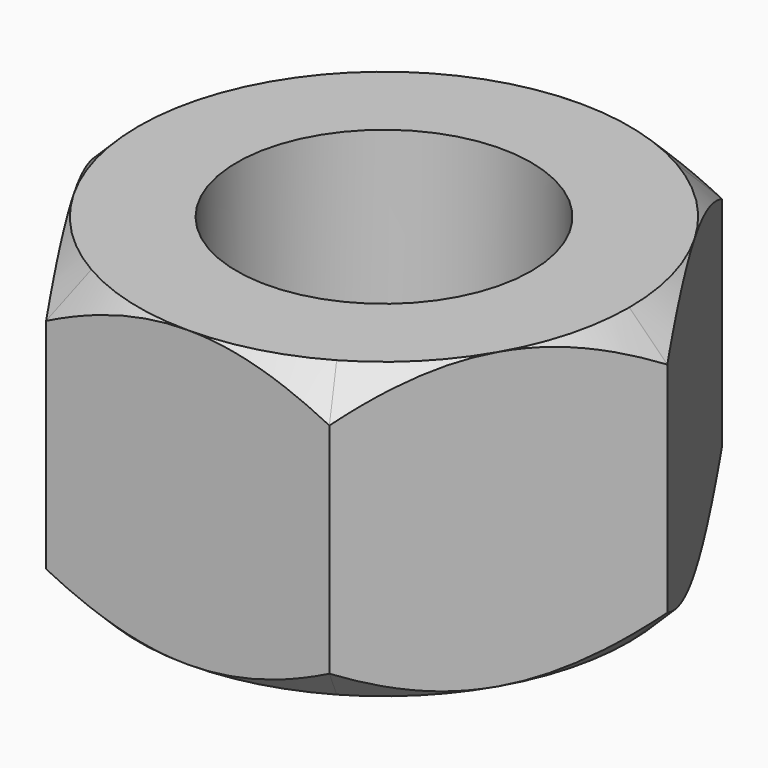
from build123d import *

# Parameters (mm, degrees)
F0_R     = 3
F1_DEPTH = 6
F2_SIZE  = 0.7735
F3_DEPTH = 6.001


# Not quite as in the source:
# - a feature names something its author has since deleted; it is built from what else it names


with BuildPart() as f1:
    # F0 (on Top) → F1 (new body)
    with BuildSketch(Plane.XY):
        Polygon((2.8867513459, 5), (-2.8867513459, 5), (-5.7735026919, 0), (-2.8867513459, -5), (2.8867513459, -5), (5.7735026919, 0), align=None)
        Circle(F0_R, mode=Mode.SUBTRACT)
        with BuildLine():
            Line((-5.7735026919, 0), (-2.8867513459, 5))
            ThreePointArc((-2.8867513459, 5), (-5, 2.8867513459), (-5.7735026919, 0))
        make_face()
        with BuildLine():
            Line((-2.8867513459, -5), (-5.7735026919, 0))
            ThreePointArc((-5.7735026919, 0), (-5, -2.8867513459), (-2.8867513459, -5))
        make_face()
        with BuildLine():
            ThreePointArc((2.8867513459, -5), (5, -2.8867513459), (5.7735026919, 0))
            Line((5.7735026919, 0), (2.8867513459, -5))
        make_face()
        with BuildLine():
            ThreePointArc((5.7735026919, 0), (5, 2.8867513459), (2.8867513459, 5))
            Line((2.8867513459, 5), (5.7735026919, 0))
        make_face()
        with BuildLine():
            ThreePointArc((2.8867513459, 5), (0, 5.7735026919), (-2.8867513459, 5))
            Line((-2.8867513459, 5), (2.8867513459, 5))
        make_face()
        with BuildLine():
            Line((2.8867513459, -5), (-2.8867513459, -5))
            ThreePointArc((-2.8867513459, -5), (0, -5.7735026919), (2.8867513459, -5))
        make_face()
    extrude(amount=F1_DEPTH)

    # F2
    f2_edges = [f1.edges().sort_by_distance(p)[0] for p in [
        (2.886751, 5, 6),
        (2.886751, 5, 0),
    ]]
    chamfer(f2_edges, length=F2_SIZE)

    # F0 (on Top) → F3 (cut, through all)
    with BuildSketch(Plane.XY):
        with BuildLine():
            Line((-2.8867513459, -5), (-5.7735026919, 0))
            ThreePointArc((-5.7735026919, 0), (-5, -2.8867513459), (-2.8867513459, -5))
        make_face()
        with BuildLine():
            Line((-5.7735026919, 0), (-2.8867513459, 5))
            ThreePointArc((-2.8867513459, 5), (-5, 2.8867513459), (-5.7735026919, 0))
        make_face()
        with BuildLine():
            ThreePointArc((2.8867513459, 5), (0, 5.7735026919), (-2.8867513459, 5))
            Line((-2.8867513459, 5), (2.8867513459, 5))
        make_face()
        with BuildLine():
            ThreePointArc((5.7735026919, 0), (5, 2.8867513459), (2.8867513459, 5))
            Line((2.8867513459, 5), (5.7735026919, 0))
        make_face()
        with BuildLine():
            ThreePointArc((2.8867513459, -5), (5, -2.8867513459), (5.7735026919, 0))
            Line((5.7735026919, 0), (2.8867513459, -5))
        make_face()
        with BuildLine():
            Line((2.8867513459, -5), (-2.8867513459, -5))
            ThreePointArc((-2.8867513459, -5), (0, -5.7735026919), (2.8867513459, -5))
        make_face()
    extrude(amount=F3_DEPTH, mode=Mode.SUBTRACT)


solid = f1.part
